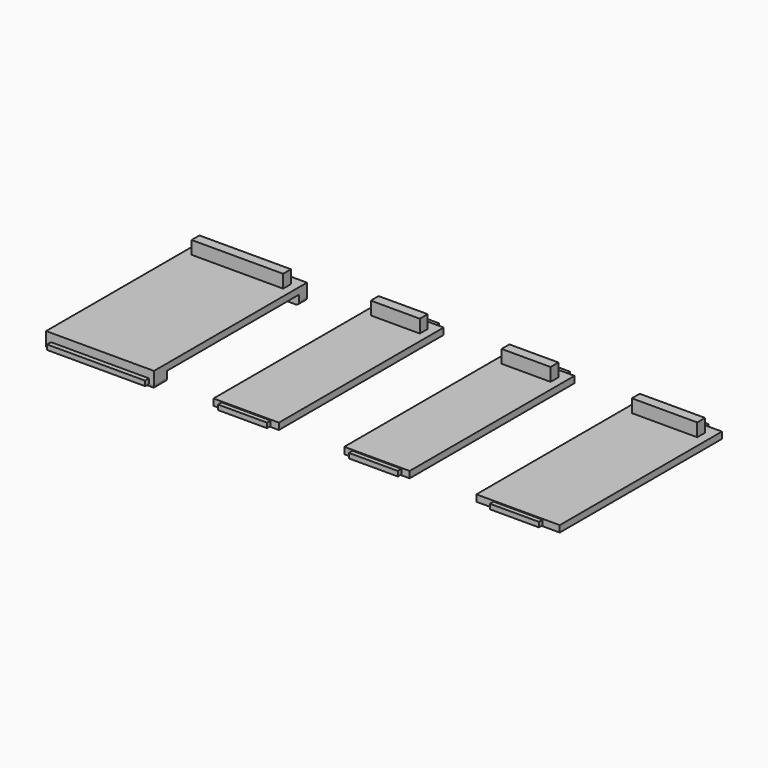
from build123d import *

# Parameters (mm, degrees)
F0_W          = 15
F0_H          = 1.4
F1_DEPTH      = 0.75
F0_W_2        = 28
F0_H_2        = 3
F2_DEPTH      = 1
F0_W_3        = 20
F3_DEPTH      = 5
F3_DEPTH_BACK = 1.5
F4_W          = 23
F4_H          = 2
F5_DEPTH      = 0.5
F6_W          = 13
F6_H          = 1.5
F7_DEPTH      = 0.5
F8_W          = 16
F8_H          = 1.5
F9_DEPTH      = 0.5
F10_W         = 33
F10_H         = 5
F11_DEPTH     = 3
F12_W         = 30
F12_H         = 1.5
F13_DEPTH     = 1.5
F14_W         = 30
F14_H         = 1.5
F15_DEPTH     = 1.5
F16_R         = 0.99999


# Not quite as in the source:
# - a fillet or chamfer is up to 0.001 mm smaller than in the source, because OpenCascade refuses the exact size
# - a feature names something its author has since deleted; it is built from what else it names


with BuildPart() as f1:
    # F0 (on Top) → F1 (new body, symmetric)
    with BuildSketch(Plane.XY):
        with Locations((-20, 32.2)):
            Rectangle(F0_W, F0_H)
    extrude(amount=F1_DEPTH, both=True)



with BuildPart() as f1b:
    # F0 (on Top) → F1, piece 2 (new body, symmetric)
    with BuildSketch(Plane.XY):
        with Locations((20, 32.2)):
            Rectangle(F0_W, F0_H)
    extrude(amount=F1_DEPTH, both=True)



with BuildPart() as f1c:
    # F0 (on Top) → F1, piece 3 (new body, symmetric)
    with BuildSketch(Plane.XY):
        with Locations((62.75, 31.7)):
            Rectangle(F0_W, F0_H)
    extrude(amount=F1_DEPTH, both=True)



with BuildPart() as f1d:
    # F0 (on Top) → F1, piece 4 (new body, symmetric)
    with BuildSketch(Plane.XY):
        with Locations((62.75, -31.7)):
            Rectangle(F0_W, F0_H)
    extrude(amount=F1_DEPTH, both=True)


with BuildPart() as f1e:
    # F0 (on Top) → F1, piece 5 (new body, symmetric)
    with BuildSketch(Plane.XY):
        with Locations((20, -32.2)):
            Rectangle(F0_W, F0_H)
    extrude(amount=F1_DEPTH, both=True)


with BuildPart() as f1f:
    # F0 (on Top) → F1, piece 6 (new body, symmetric)
    with BuildSketch(Plane.XY):
        with Locations((-20, -32.2)):
            Rectangle(F0_W, F0_H)
    extrude(amount=F1_DEPTH, both=True)


with BuildPart() as f2:
    # F0 (on Top) → F2 (new body, symmetric)
    with BuildSketch(Plane.XY):
        Polygon((-50, 29.25), (-83, 29.25), (-83, -29.25), (-76, -29.25), (-57, -29.25), (-50, -29.25), align=None)
        with Locations((-66.5, 24.75)):
            Rectangle(F0_W_2, F0_H_2, mode=Mode.SUBTRACT)
    extrude(amount=F2_DEPTH, both=True)

    # F0 (on Top) → F3 (join, two sides)
    with BuildSketch(Plane.XY) as f3_sk:
        with Locations((-66.5, 24.75)):
            Rectangle(F0_W_2, F0_H_2)
    extrude(amount=F3_DEPTH)
    extrude(f3_sk.sketch, amount=-F3_DEPTH_BACK)

    # F4 (on face) → F5 (cut)
    with BuildSketch(Plane(origin=(0, 26.25, 0), x_dir=(-1, 0, 0), z_dir=(0, 1, 0))):
        with Locations((66.5, 3.5)):
            Rectangle(F4_W, F4_H)
    extrude(amount=-F5_DEPTH, mode=Mode.SUBTRACT)

    # F10 (on face) → F11 (join)
    with BuildSketch(Plane(origin=(0, 0, -1), x_dir=(1, 0, 0), z_dir=(0, 0, -1))):
        Polygon((-83, -26.25), (-83, -29.25), (-50, -29.25), (-50, -26.25), (-52.5, -26.25), (-80.5, -26.25), align=None)
        with Locations((-66.5, 26.75)):
            Rectangle(F10_W, F10_H)
    extrude(amount=F11_DEPTH)

    # F12 (on face) → F13 (join)
    with BuildSketch(Plane(origin=(0, 29.25, 0), x_dir=(-1, 0, 0), z_dir=(0, 1, 0))):
        with Locations((66.5, -2.25)):
            Rectangle(F12_W, F12_H)
    extrude(amount=F13_DEPTH)

    # F14 (on face) → F15 (join)
    with BuildSketch(Plane.XZ.offset(29.25)):
        with Locations((-66.5, -2.25)):
            Rectangle(F14_W, F14_H)
    extrude(amount=F15_DEPTH)

    # F16 (radius 1 in the source; OpenCascade refuses exactly that, so slightly less here)
    f16_edges = [f2.edges().sort_by_distance(p)[0] for p in [
        (-66.5, 29.25, -4),
        (-66.5, -29.25, -4),
        (-83, 27.75, -4),
        (-83, -26.75, -4),
        (-50, 27.75, -4),
        (-50, -26.75, -4),
    ]]
    fillet(f16_edges, radius=F16_R)


with BuildPart() as f1_1:
    add(f1.part)

    add(f1f.part)  # F2#2 merges F1f
    # F0 (on Top) → F2, piece 2 (join, symmetric)
    with BuildSketch(Plane.XY):
        Polygon((-27.5, 31.5), (-30, 31.5), (-30, -31.5), (-27.5, -31.5), (-12.5, -31.5), (-10, -31.5), (-10, 31.5), (-12.5, 31.5), align=None)
        with Locations((-20, 27)):
            Rectangle(F0_W, F0_H_2, mode=Mode.SUBTRACT)
    extrude(amount=F2_DEPTH, both=True)

    # F0 (on Top) → F3, piece 2 (join, two sides)
    with BuildSketch(Plane.XY) as f3_2_sk:
        with Locations((-20, 27)):
            Rectangle(F0_W, F0_H_2)
    extrude(amount=F3_DEPTH)
    extrude(f3_2_sk.sketch, amount=-F3_DEPTH_BACK)


with BuildPart() as f1b_1:
    add(f1b.part)

    add(f1e.part)  # F2#3 merges F1e
    # F0 (on Top) → F2, piece 3 (join, symmetric)
    with BuildSketch(Plane.XY):
        Polygon((12.5, 31.5), (10, 31.5), (10, -31.5), (12.5, -31.5), (27.5, -31.5), (30, -31.5), (30, 31.5), (27.5, 31.5), align=None)
        with Locations((20, 27)):
            Rectangle(F0_W, F0_H_2, mode=Mode.SUBTRACT)
    extrude(amount=F2_DEPTH, both=True)

    # F0 (on Top) → F3, piece 3 (join, two sides)
    with BuildSketch(Plane.XY) as f3_3_sk:
        with Locations((20, 27)):
            Rectangle(F0_W, F0_H_2)
    extrude(amount=F3_DEPTH)
    extrude(f3_3_sk.sketch, amount=-F3_DEPTH_BACK)


with BuildPart() as f1c_1:
    add(f1c.part)

    add(f1d.part)  # F2#4 merges F1d
    # F0 (on Top) → F2, piece 4 (join, symmetric)
    with BuildSketch(Plane.XY):
        Polygon((55.25, 31), (50, 31), (50, -31), (55.25, -31), (70.25, -31), (75.5, -31), (75.5, 31), (70.25, 31), align=None)
        with Locations((62.75, 26.5)):
            Rectangle(F0_W_3, F0_H_2, mode=Mode.SUBTRACT)
    extrude(amount=F2_DEPTH, both=True)

    # F0 (on Top) → F3, piece 4 (join, two sides)
    with BuildSketch(Plane.XY) as f3_4_sk:
        with Locations((62.75, 26.5)):
            Rectangle(F0_W_3, F0_H_2)
    extrude(amount=F3_DEPTH)
    extrude(f3_4_sk.sketch, amount=-F3_DEPTH_BACK)

    # F8 (on face) → F9 (cut)
    with BuildSketch(Plane(origin=(0, 28, 0), x_dir=(-1, 0, 0), z_dir=(0, 1, 0))):
        with Locations((-62.75, 3.75)):
            Rectangle(F8_W, F8_H)
    extrude(amount=-F9_DEPTH, mode=Mode.SUBTRACT)


with BuildPart() as f7_tool:
    # F6 (on face) → F7 (new body)
    with BuildSketch(Plane(origin=(0, 28.5, 0), x_dir=(-1, 0, 0), z_dir=(0, 1, 0))):
        with Locations((-20, 3.75)):
            Rectangle(F6_W, F6_H)
        with Locations((20, 3.75)):
            Rectangle(F6_W, F6_H)
    extrude(amount=-F7_DEPTH)


with BuildPart() as f1_2:
    add(f1_1.part)

    # F7: cut by f7_tool
    add(f7_tool.part, mode=Mode.SUBTRACT)


with BuildPart() as f1b_2:
    add(f1b_1.part)

    # F7: cut by f7_tool
    add(f7_tool.part, mode=Mode.SUBTRACT)


solid = Compound([f2.part, f1c_1.part, f1_2.part, f1b_2.part])
